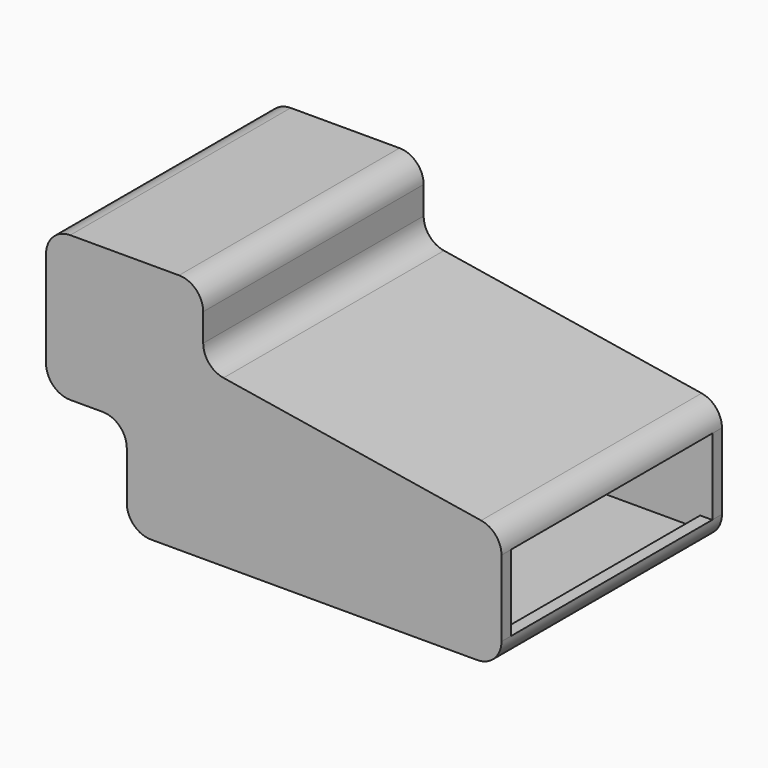
from build123d import *

# Parameters (mm, degrees)
F1_DEPTH = 57.912
F2_R     = 5.08
F3_T     = -2.54


# Not quite as in the source:
# - a shell that OpenCascade refuses in one call is made with other operations: the cavity is built on its own and cut out


with BuildPart() as f1:
    # F0 (on Front) → F1 (new body)
    with BuildSketch(Plane.XZ):
        Polygon((-7.2342143664, 44.1616670006), (-40.2542143664, 44.1616670006), (-40.2542143664, 13.6816670006), (-23.2922839558, 13.6816670006), (-23.2922839558, -6.6383329994), (55.4477160442, -6.6383329994), (55.4477160442, 18.7616670006), (-7.2342143664, 28.9216670006), align=None)
    extrude(amount=F1_DEPTH)

    # F2
    f2_edges = [f1.edges().sort_by_distance(p)[0] for p in [
        (-7.234214, -28.956, 44.161667),
        (-7.234214, -28.956, 28.921667),
        (55.447716, -28.956, 18.761667),
        (55.447716, -28.956, -6.638333),
        (-40.254214, -28.956, 44.161667),
        (-40.254214, -28.956, 13.681667),
        (-23.292284, -28.956, 13.681667),
        (-23.292284, -28.956, -6.638333),
    ]]
    fillet(f2_edges, radius=F2_R)

    # F3: a shell. OpenCascade refuses it in one call, so the cavity is built on its own and cut out:
    # the body offset inwards by the wall thickness, plus a prism from it out through each open face.
    f3_core = offset(f1.part, amount=F3_T, mode=Mode.PRIVATE)
    f3_exits = [f3_core.faces().sort_by_distance(p)[0] for p in [
        (52.907716, -28.956, 6.440221),
    ]]
    add(f3_core, mode=Mode.SUBTRACT)
    extrude(f3_exits, amount=-F3_T, mode=Mode.SUBTRACT)


solid = f1.part
